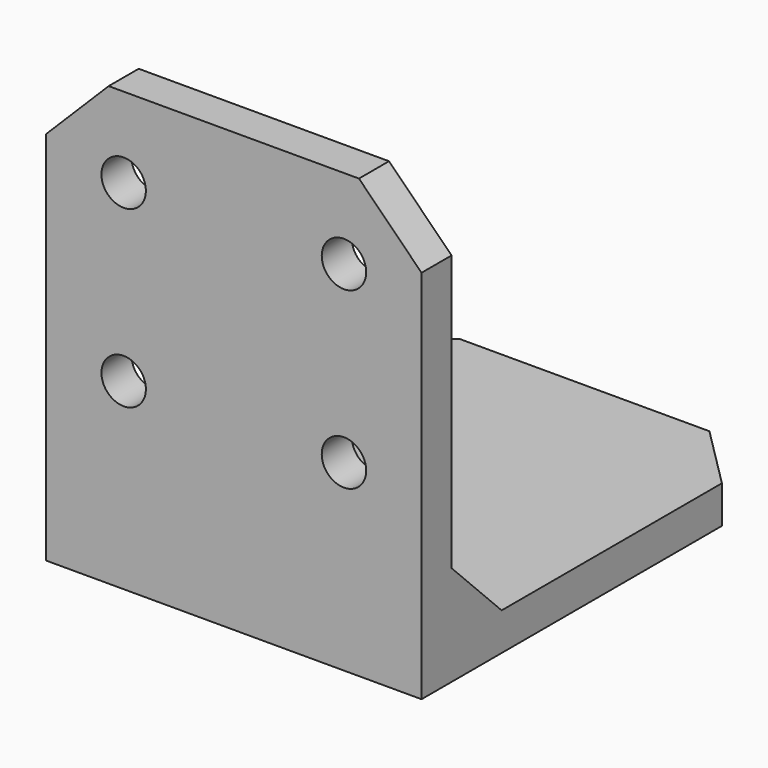
from build123d import *

# Parameters (mm, degrees)
F1_DEPTH      = 15
F1_DEPTH_BACK = 15
F2_R          = 1.775
F3_DEPTH      = 25
F4_W          = 5
F4_H          = 5
F5_DEPTH      = 15
F5_DEPTH_BACK = 15
F6_SIZE       = 4.99999
F7_SIZE       = 5
F8_SIZE       = 5
F9_SIZE       = 5
F10_SIZE      = 5


# Not quite as in the source:
# - a fillet or chamfer is up to 0.001 mm smaller than in the source, because OpenCascade refuses the exact size


with BuildPart() as f1:
    # F0 (on Right) → F1 (new body, two sides)
    with BuildSketch(Plane.YZ) as f1_sk:
        Polygon((-23.8343827544, 11.557416933), (-26.8343827544, 11.557416933), (-26.8343827544, -23.442583067), (8.1656172456, -23.442583067), (8.1656172456, -20.442583067), (-23.8343827544, -20.442583067), align=None)
    extrude(amount=F1_DEPTH)
    extrude(f1_sk.sketch, amount=-F1_DEPTH_BACK)

    # F2 (on face) → F3 (cut)
    with BuildSketch(Plane(origin=(0, -23.8343827544, 0), x_dir=(-1, 0, 0), z_dir=(0, 1, 0))):
        with Locations((-8.8, 5.157416933)):
            Circle(F2_R)
        with Locations((8.8, 5.157416933)):
            Circle(F2_R)
        with Locations((8.8, -8.8)):
            Circle(F2_R)
        with Locations((-8.8, -8.8)):
            Circle(F2_R)
    extrude(amount=-F3_DEPTH, mode=Mode.SUBTRACT)

    # F4 (on Right) → F5 (join, two sides)
    with BuildSketch(Plane.YZ) as f5_sk:
        with Locations((-21.3343827544, -17.942583067)):
            Rectangle(F4_W, F4_H)
    extrude(amount=F5_DEPTH)
    extrude(f5_sk.sketch, amount=-F5_DEPTH_BACK)

    # F6 (size 5 in the source; OpenCascade refuses exactly that, so slightly less here)
    f6_edges = [f1.edges().sort_by_distance(p)[0] for p in [
        (0, -18.834383, -15.442583),
    ]]
    chamfer(f6_edges, length=F6_SIZE)

    # F7
    f7_edges = [f1.edges().sort_by_distance(p)[0] for p in [
        (-15, -25.334383, 11.557417),
    ]]
    chamfer(f7_edges, length=F7_SIZE)

    # F8
    f8_edges = [f1.edges().sort_by_distance(p)[0] for p in [
        (15, -25.334383, 11.557417),
    ]]
    chamfer(f8_edges, length=F8_SIZE)

    # F9
    f9_edges = [f1.edges().sort_by_distance(p)[0] for p in [
        (15, 8.165617, -21.942583),
    ]]
    chamfer(f9_edges, length=F9_SIZE)

    # F10
    f10_edges = [f1.edges().sort_by_distance(p)[0] for p in [
        (-15, 8.165617, -21.942583),
    ]]
    chamfer(f10_edges, length=F10_SIZE)


solid = f1.part
